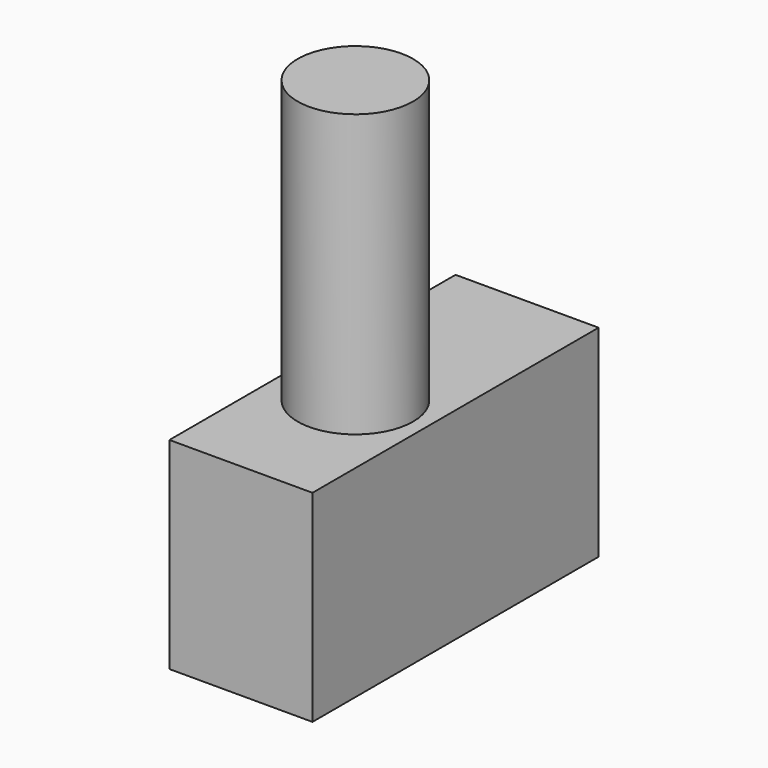
from build123d import *

# Parameters (mm, degrees)
F0_W     = 25.4
F0_H     = 25.4
F1_DEPTH = 25.4
F2_DEPTH = 38.1
F3_DEPTH = 10.414
F4_R     = 10.2474826173
F5_DEPTH = 73.152


# Not quite as in the source:
# - the program builds the solid bodies; features that only make, move or delete a surface that nothing else refers to are left out


with BuildPart() as f1:
    # F0 (on Front) → F1 (new body)
    with BuildSketch(Plane.XZ):
        Rectangle(F0_W, F0_H)
    extrude(amount=F1_DEPTH)

    # F2 (add): a face of the model
    f2_faces = [f1.faces().sort_by_distance(p)[0] for p in [
        (0, 0, 0),
    ]]
    extrude(f2_faces, amount=F2_DEPTH)

    # F3 (add): a face of the model
    f3_faces = [f1.faces().sort_by_distance(p)[0] for p in [
        (0, 6.35, 12.7),
    ]]
    extrude(f3_faces, amount=F3_DEPTH)

    # F4 (on Top) → F5 (join)
    with BuildSketch(Plane.XY):
        Circle(F4_R)
    extrude(amount=F5_DEPTH)


solid = f1.part
